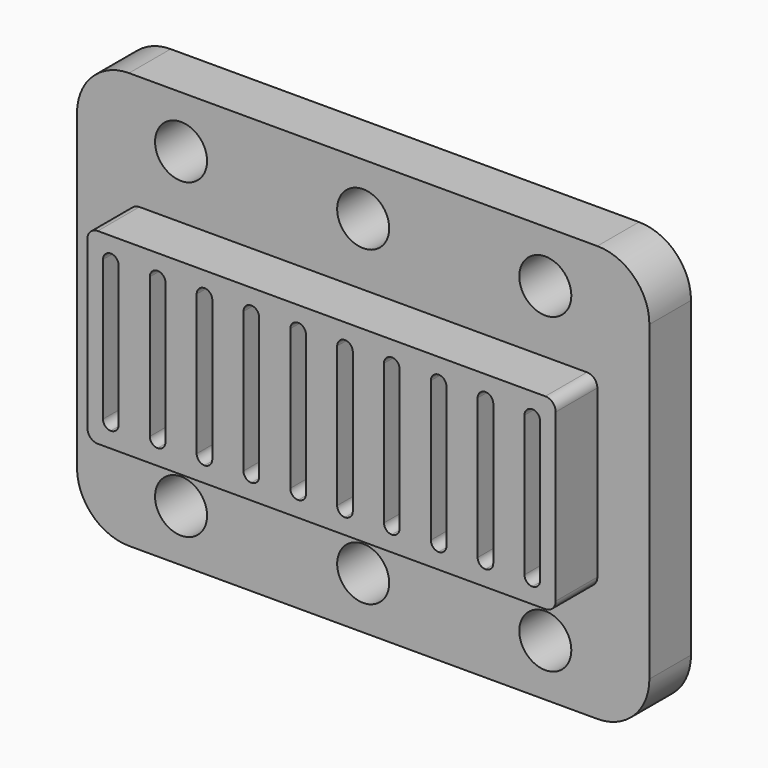
from build123d import *

# Parameters (mm, degrees)
F0_R         = 2.5
F1_DEPTH     = 5
F2_TEXT_SIZE = 9.0070198187
F3_DEPTH     = 1
F5_DEPTH     = 5


# Not quite as in the source:
# - Text() gives the source's letters only with a copy of the font that has no kerning and outlines rounded to 1/6400 em; it was checked with that copy


with BuildPart() as f1:
    # F0 (on Front) → F1 (new body)
    with BuildSketch(Plane.XZ):
        with BuildLine():
            Line((-50, 0), (-5, 0))
            ThreePointArc((-5, 0), (-1.4644660941, 1.4644660941), (0, 5))
            Line((0, 5), (0, 35))
            ThreePointArc((0, 35), (-1.4644660941, 38.5355339059), (-5, 40))
            Line((-5, 40), (-50, 40))
            ThreePointArc((-50, 40), (-53.5355339059, 38.5355339059), (-55, 35))
            Line((-55, 35), (-55, 5))
            ThreePointArc((-55, 5), (-53.5355339059, 1.4644660941), (-50, 0))
        make_face()
        with Locations((-45, 5)):
            Circle(F0_R, mode=Mode.SUBTRACT)
        with Locations((-27.5, 5)):
            Circle(F0_R, mode=Mode.SUBTRACT)
        with Locations((-10, 5)):
            Circle(F0_R, mode=Mode.SUBTRACT)
        with Locations((-45, 35)):
            Circle(F0_R, mode=Mode.SUBTRACT)
        with Locations((-27.5, 35)):
            Circle(F0_R, mode=Mode.SUBTRACT)
        with Locations((-10, 35)):
            Circle(F0_R, mode=Mode.SUBTRACT)
    extrude(amount=F1_DEPTH)

    # F2 (on face) → F3 (join)
    with BuildSketch(Plane(origin=(0, 0, 0), x_dir=(-1, 0, 0), z_dir=(0, 1, 0))):
        with Locations((15.642057173, 17.4909178168)):
            Text('Merlin', F2_TEXT_SIZE, font='Open Sans', text_align=(TextAlign.LEFT, TextAlign.BOTTOM))
    extrude(amount=F3_DEPTH)

    # F4 (on face) → F5 (join)
    with BuildSketch(Plane.XZ.offset(5)):
        with BuildLine():
            Line((-6, 29), (-49, 29))
            ThreePointArc((-49, 29), (-49.7071067812, 28.7071067812), (-50, 28))
            Line((-50, 28), (-50, 12))
            ThreePointArc((-50, 12), (-49.7071067812, 11.2928932188), (-49, 11))
            Line((-49, 11), (-6, 11))
            ThreePointArc((-6, 11), (-5.2928932188, 11.2928932188), (-5, 12))
            Line((-5, 12), (-5, 28))
            ThreePointArc((-5, 28), (-5.2928932188, 28.7071067812), (-6, 29))
        make_face()
        with BuildLine():
            Line((-48.5, 13.25), (-48.5, 26.75))
            ThreePointArc((-48.5, 26.75), (-48.2803300859, 27.2803300859), (-47.75, 27.5))
            ThreePointArc((-47.75, 27.5), (-47.2196699141, 27.2803300859), (-47, 26.75))
            Line((-47, 26.75), (-47, 13.25))
            ThreePointArc((-47, 13.25), (-47.2196699141, 12.7196699141), (-47.75, 12.5))
            ThreePointArc((-47.75, 12.5), (-48.2803300859, 12.7196699141), (-48.5, 13.25))
        make_face(mode=Mode.SUBTRACT)
        with BuildLine():
            Line((-44, 13.25), (-44, 26.75))
            ThreePointArc((-44, 26.75), (-43.7803300859, 27.2803300859), (-43.25, 27.5))
            ThreePointArc((-43.25, 27.5), (-42.7196699141, 27.2803300859), (-42.5, 26.75))
            Line((-42.5, 26.75), (-42.5, 13.25))
            ThreePointArc((-42.5, 13.25), (-42.7196699141, 12.7196699141), (-43.25, 12.5))
            ThreePointArc((-43.25, 12.5), (-43.7803300859, 12.7196699141), (-44, 13.25))
        make_face(mode=Mode.SUBTRACT)
        with BuildLine():
            Line((-39.5, 13.25), (-39.5, 26.75))
            ThreePointArc((-39.5, 26.75), (-39.2803300859, 27.2803300859), (-38.75, 27.5))
            ThreePointArc((-38.75, 27.5), (-38.2196699141, 27.2803300859), (-38, 26.75))
            Line((-38, 26.75), (-38, 13.25))
            ThreePointArc((-38, 13.25), (-38.2196699141, 12.7196699141), (-38.75, 12.5))
            ThreePointArc((-38.75, 12.5), (-39.2803300859, 12.7196699141), (-39.5, 13.25))
        make_face(mode=Mode.SUBTRACT)
        with BuildLine():
            Line((-35, 13.25), (-35, 26.75))
            ThreePointArc((-35, 26.75), (-34.7803300859, 27.2803300859), (-34.25, 27.5))
            ThreePointArc((-34.25, 27.5), (-33.7196699141, 27.2803300859), (-33.5, 26.75))
            Line((-33.5, 26.75), (-33.5, 13.25))
            ThreePointArc((-33.5, 13.25), (-33.7196699141, 12.7196699141), (-34.25, 12.5))
            ThreePointArc((-34.25, 12.5), (-34.7803300859, 12.7196699141), (-35, 13.25))
        make_face(mode=Mode.SUBTRACT)
        with BuildLine():
            Line((-30.5, 13.25), (-30.5, 26.75))
            ThreePointArc((-30.5, 26.75), (-30.2803300859, 27.2803300859), (-29.75, 27.5))
            ThreePointArc((-29.75, 27.5), (-29.2196699141, 27.2803300859), (-29, 26.75))
            Line((-29, 26.75), (-29, 13.25))
            ThreePointArc((-29, 13.25), (-29.2196699141, 12.7196699141), (-29.75, 12.5))
            ThreePointArc((-29.75, 12.5), (-30.2803300859, 12.7196699141), (-30.5, 13.25))
        make_face(mode=Mode.SUBTRACT)
        with BuildLine():
            Line((-26, 13.25), (-26, 26.75))
            ThreePointArc((-26, 26.75), (-25.7803300859, 27.2803300859), (-25.25, 27.5))
            ThreePointArc((-25.25, 27.5), (-24.7196699141, 27.2803300859), (-24.5, 26.75))
            Line((-24.5, 26.75), (-24.5, 13.25))
            ThreePointArc((-24.5, 13.25), (-24.7196699141, 12.7196699141), (-25.25, 12.5))
            ThreePointArc((-25.25, 12.5), (-25.7803300859, 12.7196699141), (-26, 13.25))
        make_face(mode=Mode.SUBTRACT)
        with BuildLine():
            Line((-21.5, 13.25), (-21.5, 26.75))
            ThreePointArc((-21.5, 26.75), (-21.2803300859, 27.2803300859), (-20.75, 27.5))
            ThreePointArc((-20.75, 27.5), (-20.2196699141, 27.2803300859), (-20, 26.75))
            Line((-20, 26.75), (-20, 13.25))
            ThreePointArc((-20, 13.25), (-20.2196699141, 12.7196699141), (-20.75, 12.5))
            ThreePointArc((-20.75, 12.5), (-21.2803300859, 12.7196699141), (-21.5, 13.25))
        make_face(mode=Mode.SUBTRACT)
        with BuildLine():
            Line((-17, 13.25), (-17, 26.75))
            ThreePointArc((-17, 26.75), (-16.7803300859, 27.2803300859), (-16.25, 27.5))
            ThreePointArc((-16.25, 27.5), (-15.7196699141, 27.2803300859), (-15.5, 26.75))
            Line((-15.5, 26.75), (-15.5, 13.25))
            ThreePointArc((-15.5, 13.25), (-15.7196699141, 12.7196699141), (-16.25, 12.5))
            ThreePointArc((-16.25, 12.5), (-16.7803300859, 12.7196699141), (-17, 13.25))
        make_face(mode=Mode.SUBTRACT)
        with BuildLine():
            Line((-12.5, 13.25), (-12.5, 26.75))
            ThreePointArc((-12.5, 26.75), (-12.2803300859, 27.2803300859), (-11.75, 27.5))
            ThreePointArc((-11.75, 27.5), (-11.2196699141, 27.2803300859), (-11, 26.75))
            Line((-11, 26.75), (-11, 13.25))
            ThreePointArc((-11, 13.25), (-11.2196699141, 12.7196699141), (-11.75, 12.5))
            ThreePointArc((-11.75, 12.5), (-12.2803300859, 12.7196699141), (-12.5, 13.25))
        make_face(mode=Mode.SUBTRACT)
        with BuildLine():
            Line((-8, 13.25), (-8, 26.75))
            ThreePointArc((-8, 26.75), (-7.7803300859, 27.2803300859), (-7.25, 27.5))
            ThreePointArc((-7.25, 27.5), (-6.7196699141, 27.2803300859), (-6.5, 26.75))
            Line((-6.5, 26.75), (-6.5, 13.25))
            ThreePointArc((-6.5, 13.25), (-6.7196699141, 12.7196699141), (-7.25, 12.5))
            ThreePointArc((-7.25, 12.5), (-7.7803300859, 12.7196699141), (-8, 13.25))
        make_face(mode=Mode.SUBTRACT)
    extrude(amount=F5_DEPTH)


solid = f1.part
